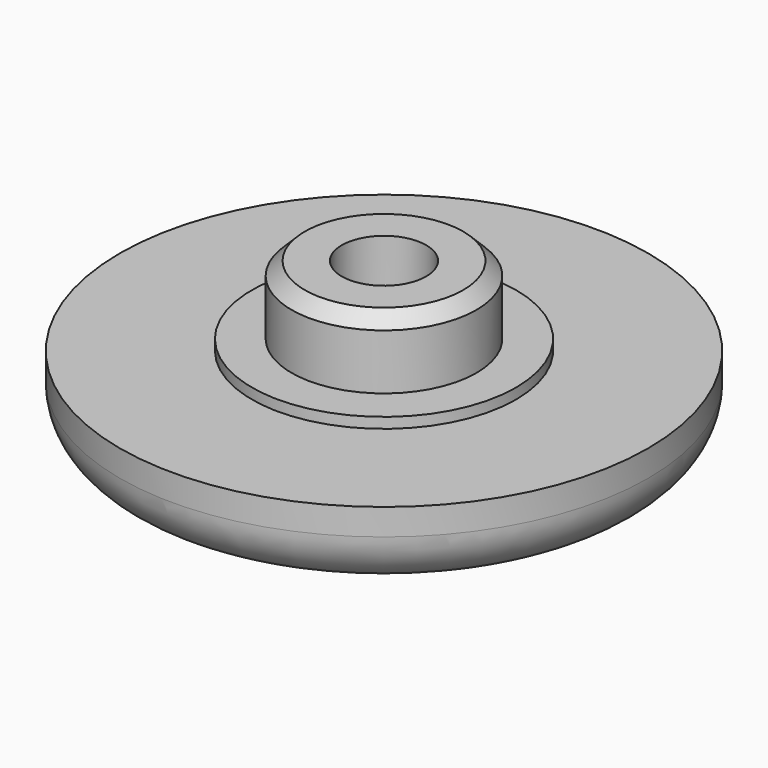
from build123d import *

# Parameters (mm, degrees)
F2_SIZE  = 0.5
F3_R     = 5
F3_R_2   = 3.5
F4_DEPTH = 0.4
F5_R     = 2
F6_R     = 1.6
F7_DEPTH = 25
F8_R     = 3
F8_R_2   = 1.6
F9_DEPTH = 2.5


# Not quite as in the source:
# - a feature names something its author has since deleted; it is built from what else it names


with BuildPart() as f1:
    # F0 (on Front) → F1 (revolve)
    with BuildSketch(Plane.XZ):
        Polygon((3.5, 6), (0, 6), (0, 0), (10, 0), (10, 3), (3.5, 3), align=None)
    revolve(axis=Axis((0, 0, 3), (0, 0, -1)))

    # F2
    f2_edges = [f1.edges().sort_by_distance(p)[0] for p in [
        (-3.5, 0, 6),
    ]]
    chamfer(f2_edges, length=F2_SIZE)

    # F3 (on face) → F4 (join)
    with BuildSketch(Plane.XY.offset(3)):
        Circle(F3_R)
        Circle(F3_R_2, mode=Mode.SUBTRACT)
    extrude(amount=F4_DEPTH)

    # F5
    f5_edges = [f1.edges().sort_by_distance(p)[0] for p in [
        (-10, 0, 0),
    ]]
    fillet(f5_edges, radius=F5_R)

    # F6 (on face) → F7 (cut)
    with BuildSketch(Plane.XY.offset(6)):
        Circle(F6_R)
    extrude(amount=-F7_DEPTH, mode=Mode.SUBTRACT)

    # F8 (on face) → F9 (cut)
    with BuildSketch(Plane(origin=(0, 0, 0), x_dir=(1, 0, 0), z_dir=(0, 0, -1))):
        Circle(F8_R)
        Circle(F8_R_2, mode=Mode.SUBTRACT)
    extrude(amount=-F9_DEPTH, mode=Mode.SUBTRACT)


solid = f1.part
